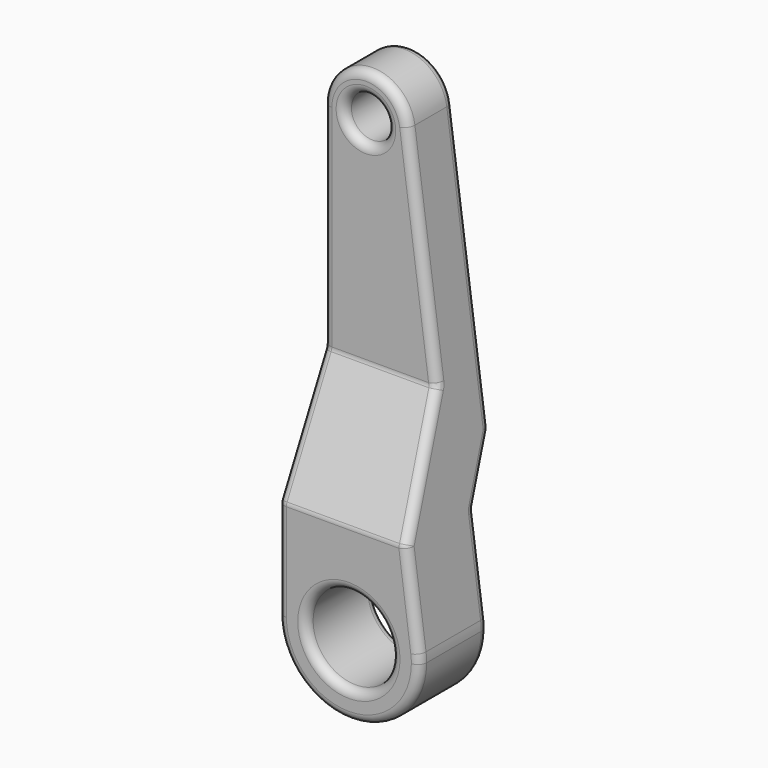
from build123d import *

# Parameters (mm, degrees)
F1_DEPTH = 40
F3_DEPTH = 50.001
F4_R     = 7.5
F4_R_2   = 15
F5_DEPTH = 40.001
F6_T     = -8
F8_DEPTH = 14
F9_R     = 3


with BuildPart() as f1:
    # F0 (on Front) → F1 (new body)
    with BuildSketch(Plane.XZ):
        with BuildLine():
            ThreePointArc((-25, 0), (0, -25), (25, 0))
            ThreePointArc((25, 0), (24.9446289464, 1.6629752631), (24.7787610619, 3.3185840708))
            ThreePointArc((24.7787610619, 3.3185840708), (-1.6629752631, 24.9446289464), (-25, 0))
        make_face()
        with BuildLine():
            ThreePointArc((-25, 0), (-1.6629752631, 24.9446289464), (24.7787610619, 3.3185840708))
            Line((24.7787610619, 3.3185840708), (4.8672566372, 151.9911504425))
            ThreePointArc((4.8672566372, 151.9911504425), (4.9667773678, 150.9977851579), (5, 150))
            ThreePointArc((5, 150), (-10, 135), (-25, 150))
            Line((-25, 150), (-25, 0))
        make_face()
        with BuildLine():
            ThreePointArc((5, 150), (4.9667773678, 150.9977851579), (4.8672566372, 151.9911504425))
            ThreePointArc((4.8672566372, 151.9911504425), (-10.9977851579, 164.9667773678), (-25, 150))
            ThreePointArc((-25, 150), (-10, 135), (5, 150))
        make_face()
    extrude(amount=F1_DEPTH)

    # F2 (on face) → F3 (cut, through all)
    with BuildSketch(Plane(origin=(-25, 0, 0), x_dir=(0, -1, 0), z_dir=(-1, 0, 0))):
        Polygon((40, 179.1010204973), (20, 179.1010204973), (20, 75), (40, 35), align=None)
        Polygon((10, 35), (0, 55), (0, 3.7116128951), (0, -38.6656261981), (10, -38.6656261981), align=None)
    extrude(amount=-F3_DEPTH, mode=Mode.SUBTRACT)

    # F4 (on face) → F5 (cut, through all)
    with BuildSketch(Plane(origin=(0, 0, 0), x_dir=(-1, 0, 0), z_dir=(0, 1, 0))):
        with Locations((10, 150)):
            Circle(F4_R)
        Circle(F4_R_2)
    extrude(amount=-F5_DEPTH, mode=Mode.SUBTRACT)

    # F6
    f6_openings = [f1.faces().sort_by_distance(p)[0] for p in [
        (-6.733599, 0, 102.796196),
        (-2.895022, -5.050505, 44.89899),
        (-24.218975, -10, 17.5),
    ]]
    offset(amount=F6_T, openings=f6_openings)

    # F7 (on face) → F8 (join, through all)
    with BuildSketch(Plane(origin=(0, 0, 0), x_dir=(-1, 0, 0), z_dir=(0, 1, 0))):
        Polygon((17, 77.11145618), (-6.8243585473, 77.11145618), (-7.8957871187, 69.11145618), (17, 69.11145618), align=None)
    extrude(amount=-F8_DEPTH)

    # F9
    f9_edges = [f1.edges().sort_by_distance(p)[0] for p in [
        (-5.087821, -12, 77.111456),
        (2.799081, -12, 107.166863),
        (-8.968955, -12, 134.53433),
        (-17, -12, 106.64107),
        (-25, -20, 112.5),
        (11.3622, 0, 103.495575),
        (-10.997785, 0, 164.966777),
        (-10.997785, -20, 164.966777),
        (15, -10, 0),
        (-25, -30, 55),
        (-25, -40, 17.5),
        (-25, -10, 17.5),
        (22.657238, -40, 19.159292),
        (1.662975, -40, -24.944629),
        (17.857143, -30, 55),
        (15, -40, 0),
        (1.662975, -10, -24.944629),
        (-2.5, -20, 150),
        (10.022914, -20, 113.495575),
        (-25, 0, 102.5),
        (-4.910714, -20, 75),
        (-2.232143, -40, 35),
        (-25, -5, 45),
        (-2.5, 0, 150),
        (22.657238, -10, 19.159292),
        (-17, -23, 51.111456),
        (-2.141392, -32, 33.111456),
        (-17, -21, 15.491933),
        (-17, -10, 25.245967),
        (-17, -5, 45),
        (-17, 0, 62.055728),
        (-17, 0, 106.64107),
        (-17, -6, 136.170683),
        (-17, -32, 24.301695),
        (-5.087821, 0, 77.111456),
        (13.755161, -32, 25.361465),
        (-1.226197, -6, 137.22227),
        (8.840751, 0, 62.055728),
        (2.799081, 0, 107.166863),
        (-8.968955, 0, 134.53433),
        (-17, -7, 69.111456),
        (-4.552106, 0, 69.111456),
        (-4.552106, -14, 69.111456),
        (6.824359, -6, 77.111456),
        (-17, -6, 77.111456),
        (7.895787, -7, 69.111456),
        (19.196429, -5, 45),
        (-21, 0, 55),
        (13.821429, 0, 55),
        (-21, -10, 35),
        (16.5, -10, 35),
        (13.628696, -10, 26.305737),
        (-1.529937, -10, 22.949059),
        (11.125, -5, 45),
        (10.306501, -23, 51.111456),
        (14.793106, -21, 17.611474),
        (-1.529937, -32, 22.949059),
    ]]
    fillet(f9_edges, radius=F9_R)


solid = f1.part
